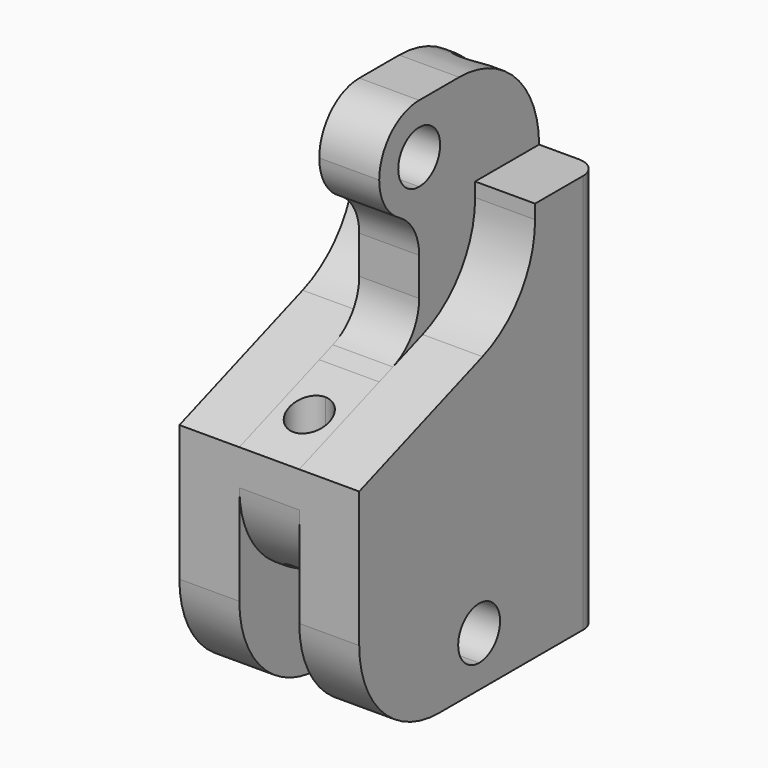
from build123d import *

# Parameters (mm, degrees)
F1_DEPTH     = 15
F3_DEPTH     = 6
F5_DEPTH     = 18
F6_R         = 10
F9_DEPTH     = 6
F10_DEPTH    = 6
F11_R        = 2
F13_DEPTH    = 6
F15_R        = 10
F19_DEPTH    = 45.001
F21_DEPTH    = 40.001
F23_DEPTH    = 6
F24_T1_DEPTH = 6


# Not quite as in the source:
# - a fillet or chamfer that OpenCascade refuses, or shapes differently, is made with other operations: its cross-section is extruded or revolved along the edge and cut away or added


with BuildPart() as f1:
    # F0 (on Front) → F1 (new body, symmetric)
    with BuildSketch(Plane.XZ):
        Polygon((9, -15), (9, 15), (3, 15), (3, 25), (-3, 25), (-3, 15), (-9, 15), (-9, -15), (-9, -25), (-3, -25), (-3, -15), (3, -15), (3, -25), (9, -25), align=None)
    extrude(amount=F1_DEPTH, both=True)

    # F2 (on face) → F3 (cut)
    with BuildSketch(Plane(origin=(-3, 0, 0), x_dir=(0, -1, 0), z_dir=(-1, 0, 0))):
        with BuildLine():
            ThreePointArc((0, 22.62), (-2.62, 20), (0, 17.38))
            Line((0, 17.38), (0, 22.62))
        make_face()
        with BuildLine():
            Line((0, 22.62), (0, 17.38))
            ThreePointArc((0, 17.38), (1.8526197667, 18.1473802333), (2.62, 20))
            ThreePointArc((2.62, 20), (1.8526197667, 21.8526197667), (0, 22.62))
        make_face()
    extrude(amount=-F3_DEPTH, mode=Mode.SUBTRACT)

    # F4 (on face) → F5 (cut)
    with BuildSketch(Plane(origin=(-9, 0, 0), x_dir=(0, -1, 0), z_dir=(-1, 0, 0))):
        with BuildLine():
            ThreePointArc((0, -22.62), (1.8526197667, -21.8526197667), (2.62, -20))
            ThreePointArc((2.62, -20), (-1.8526197667, -18.1473802333), (0, -22.62))
        make_face()
    extrude(amount=-F5_DEPTH, mode=Mode.SUBTRACT)

    # F6
    f6_edges = [f1.edges().sort_by_distance(p)[0] for p in [
        (0, 15, 25),
        (0, -15, 25),
        (6, -15, -25),
        (-6, -15, -25),
    ]]
    fillet(f6_edges, radius=F6_R)

    # F8 (on face) → F9 (cut)
    with BuildSketch(Plane(origin=(-9, 0, 0), x_dir=(0, -1, 0), z_dir=(-1, 0, 0))):
        with BuildLine():
            ThreePointArc((-7, 13.5872004348), (-5.1915204429, 7.8514360713), (-0.4202014333, 4.190274227))
            Line((-0.4202014333, 4.190274227), (15, -1.4222201011))
            Line((15, -1.4222201011), (15, 15))
            Line((15, 15), (-7, 15))
            Line((-7, 15), (-7, 13.5872004348))
        make_face()
    extrude(amount=-F9_DEPTH, mode=Mode.SUBTRACT)

    # F7 (on face) → F10 (cut)
    with BuildSketch(Plane.YZ.offset(9)):
        with BuildLine():
            Line((7, 15), (-15, 15))
            Line((-15, 15), (-15, -1.42222))
            Line((-15, -1.42222), (0.4202014333, 4.1902743281))
            ThreePointArc((0.4202014333, 4.1902743281), (5.1915204429, 7.8514361724), (7, 13.587200536))
            Line((7, 13.587200536), (7, 15))
        make_face()
    extrude(amount=-F10_DEPTH, mode=Mode.SUBTRACT)

    # F11
    f11_edges = [f1.edges().sort_by_distance(p)[0] for p in [
        (9, 15, -5),
        (-9, 15, -5),
    ]]
    fillet(f11_edges, radius=F11_R)

    # F12 (on face) → F13 (cut)
    with BuildSketch(Plane(origin=(-3, 0, 0), x_dir=(0, -1, 0), z_dir=(-1, 0, 0))):
        with BuildLine():
            Line((5, 25), (0, 25))
            ThreePointArc((0, 25), (3.5355339059, 23.5355339059), (5, 20))
            Line((5, 20), (5, 2.2174822415))
            Line((5, 2.2174822415), (15, -1.4222201011))
            Line((15, -1.4222201011), (15, 15))
            ThreePointArc((15, 15), (12.0710678119, 22.0710678119), (5, 25))
        make_face()
    extrude(amount=-F13_DEPTH, mode=Mode.SUBTRACT)

    # F15
    f15_edges = [f1.edges().sort_by_distance(p)[0] for p in [
        (0, -15, -15),
    ]]
    fillet(f15_edges, radius=F15_R)

    # F18 (on face) → F19 (cut, through all)
    with BuildSketch(Plane.XY.offset(20)):
        with BuildLine():
            ThreePointArc((2, -10), (1.4142135624, -8.5857864376), (0, -8))
            Line((0, -8), (0, -12))
            ThreePointArc((0, -12), (1.4142135624, -11.4142135624), (2, -10))
        make_face()
        with BuildLine():
            Line((0, -12), (0, -8))
            ThreePointArc((0, -8), (-2, -10), (0, -12))
        make_face()
    extrude(amount=-F19_DEPTH, mode=Mode.SUBTRACT)

    # F20 (on face) → F21 (cut, through all)
    with BuildSketch(Plane(origin=(0, 0, -15), x_dir=(1, 0, 0), z_dir=(0, 0, -1))):
        with BuildLine():
            ThreePointArc((0, -9), (-2, -11), (0, -13))
            Line((0, -13), (0, -11))
            Line((0, -11), (0, -9))
        make_face()
        with BuildLine():
            Line((0, -11), (0, -13))
            ThreePointArc((0, -13), (1.4142135624, -12.4142135624), (2, -11))
            ThreePointArc((2, -11), (1.4142135624, -9.5857864376), (0, -9))
            Line((0, -9), (0, -11))
        make_face()
    extrude(amount=-F21_DEPTH, mode=Mode.SUBTRACT)

    # F22 (on face) → F23 (cut)
    with BuildSketch(Plane.YZ.offset(3)):
        with BuildLine():
            ThreePointArc((0, 15), (-3.5355339059, 16.4644660941), (-5, 20))
            Line((-5, 20), (-5, 2.2174822415))
            Line((-5.0000000325, 2.2174823308), (0, 4.037333514))
            Line((0, 4.037333514), (0, 15))
        make_face()
    extrude(amount=-F23_DEPTH, mode=Mode.SUBTRACT)

    # F24: fillet of radius 5 on 2 edges, made by hand

    # F24_s2 → F24_t1 (join)
    with BuildSketch(Plane.YZ.offset(-3)):
        with BuildLine():
            ThreePointArc((-2.5, 15.6698729811), (-0.6698729811, 13.8397459622), (0, 11.3397459622))
            Line((0, 11.3397459622), (0, 15))
            ThreePointArc((0, 15), (-1.2940952255, 15.1703708686), (-2.5, 15.6698729811))
        make_face()
        with BuildLine():
            ThreePointArc((-3.2898992834, 2.8399081011), (-0.9042397786, 4.6704890233), (0, 7.538371205))
            Line((0, 7.538371205), (0, 4.037333514))
            Line((0, 4.037333514), (-3.2898992834, 2.8399081011))
        make_face()
    extrude(amount=F24_T1_DEPTH)


solid = f1.part
